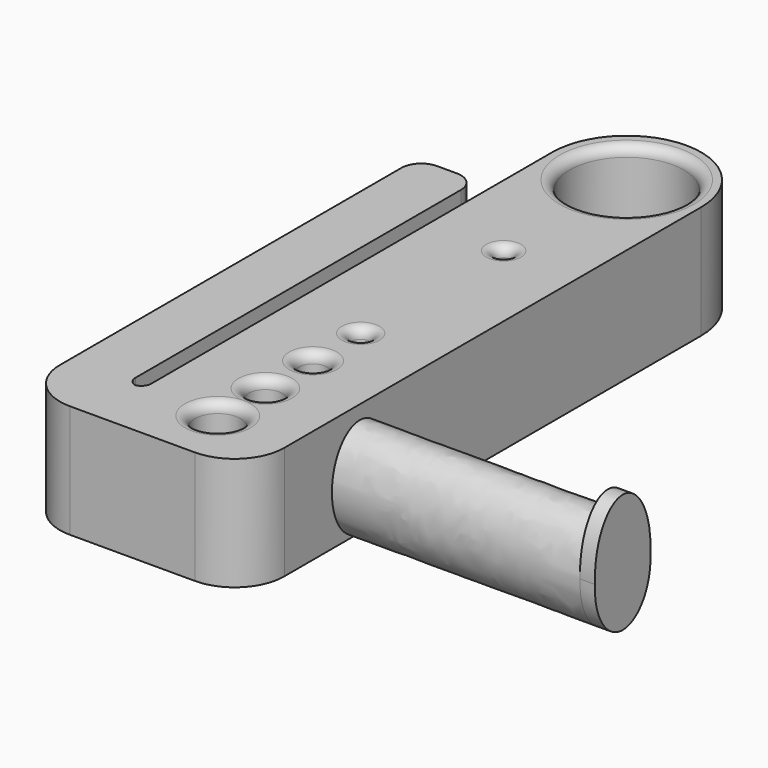
from build123d import *

# Parameters (mm, degrees)
F0_W        = 1.6
F0_H        = 6
F0_R        = 2.3
F0_R_2      = 1.7
F0_R_3      = 1.4
F0_R_4      = 0.9
F0_R_5      = 0.75
F0_R_6      = 5.75
F1_DEPTH    = 11.4
F2_R        = 5
F3_R        = 7.49999
F4_R        = 2
F5_T1_DEPTH = 11.4
F6_R        = 1
F8_DEPTH    = 25
F10_DEPTH   = 1.5


# Not quite as in the source:
# - a fillet or chamfer that OpenCascade refuses, or shapes differently, is made with other operations: its cross-section is extruded or revolved along the edge and cut away or added
# - a fillet or chamfer is up to 0.001 mm smaller than in the source, because OpenCascade refuses the exact size


with BuildPart() as f1:
    # F0 (on Top) → F1 (new body)
    with BuildSketch(Plane.XY):
        Polygon((6, 0), (0, 0), (0, -50), (6, -50), (6, -44), align=None)
        with Locations((6.8, -47)):
            Rectangle(F0_W, F0_H)
        Polygon((7.6, 15), (7.6, -44), (7.6, -50), (22.6, -50), (22.6, 15), align=None)
        with Locations((15.1, -44)):
            Circle(F0_R, mode=Mode.SUBTRACT)
        with Locations((15.1, -38)):
            Circle(F0_R_2, mode=Mode.SUBTRACT)
        with Locations((15.1, -32)):
            Circle(F0_R_3, mode=Mode.SUBTRACT)
        with Locations((15.1, -26)):
            Circle(F0_R_4, mode=Mode.SUBTRACT)
        with Locations((15.1, -8)):
            Circle(F0_R_5, mode=Mode.SUBTRACT)
        with Locations((15.1, 7.5)):
            Circle(F0_R_6, mode=Mode.SUBTRACT)
    extrude(amount=F1_DEPTH)

    # F2
    f2_edges = [f1.edges().sort_by_distance(p)[0] for p in [
        (0, -50, 5.7),
        (22.6, -50, 5.7),
    ]]
    fillet(f2_edges, radius=F2_R)

    # F3 (radius 7.5 in the source; OpenCascade refuses exactly that, so slightly less here)
    f3_edges = [f1.edges().sort_by_distance(p)[0] for p in [
        (22.6, 15, 5.7),
        (7.6, 15, 5.7),
    ]]
    fillet(f3_edges, radius=F3_R)

    # F4
    f4_edges = [f1.edges().sort_by_distance(p)[0] for p in [
        (0, 0, 5.7),
        (6, 0, 5.7),
    ]]
    fillet(f4_edges, radius=F4_R)

    # F5: fillet of radius 1 on 7 edges, made by hand

    # F5_s2 → F5_t1 (join)
    with BuildSketch(Plane.XY):
        with BuildLine():
            ThreePointArc((6, -43), (6.2928932188, -43.7071067812), (7, -44))
            Line((7, -44), (6, -44))
            Line((6, -44), (6, -43))
        make_face()
        with BuildLine():
            ThreePointArc((6.6, -44), (7.3071067812, -43.7071067812), (7.6, -43))
            Line((7.6, -43), (7.6, -44))
            Line((7.6, -44), (6.6, -44))
        make_face()
    extrude(amount=F5_T1_DEPTH)

    # F5_s3 → F5_t4 (revolve, cut)
    with BuildSketch(Plane.XZ.offset(44)):
        with BuildLine():
            ThreePointArc((17.4, 10.4), (17.6928932188, 11.1071067812), (18.4, 11.4))
            Line((18.4, 11.4), (17.4, 11.4))
            Line((17.4, 11.4), (17.4, 10.4))
        make_face()
    revolve(axis=Axis((15.1, -44, 11.4), (0, 0, 1)), mode=Mode.SUBTRACT)

    # F5_s5 → F5_t6 (revolve, cut)
    with BuildSketch(Plane.XZ.offset(38)):
        with BuildLine():
            ThreePointArc((16.8, 10.4), (17.0928932188, 11.1071067812), (17.8, 11.4))
            Line((17.8, 11.4), (16.8, 11.4))
            Line((16.8, 11.4), (16.8, 10.4))
        make_face()
    revolve(axis=Axis((15.1, -38, 11.4), (0, 0, 1)), mode=Mode.SUBTRACT)

    # F5_s7 → F5_t8 (revolve, cut)
    with BuildSketch(Plane.XZ.offset(32)):
        with BuildLine():
            ThreePointArc((16.5, 10.4), (16.7928932188, 11.1071067812), (17.5, 11.4))
            Line((17.5, 11.4), (16.5, 11.4))
            Line((16.5, 11.4), (16.5, 10.4))
        make_face()
    revolve(axis=Axis((15.1, -32, 11.4), (0, 0, 1)), mode=Mode.SUBTRACT)

    # F5_s9 → F5_t10 (revolve, cut)
    with BuildSketch(Plane.XZ.offset(26)):
        with BuildLine():
            ThreePointArc((16, 10.4), (16.2928932188, 11.1071067812), (17, 11.4))
            Line((17, 11.4), (16, 11.4))
            Line((16, 11.4), (16, 10.4))
        make_face()
    revolve(axis=Axis((15.1, -26, 11.4), (0, 0, 1)), mode=Mode.SUBTRACT)

    # F5_s11 → F5_t12 (revolve, cut)
    with BuildSketch(Plane.XZ.offset(8)):
        with BuildLine():
            ThreePointArc((15.85, 10.4), (16.1428932188, 11.1071067812), (16.85, 11.4))
            Line((16.85, 11.4), (15.85, 11.4))
            Line((15.85, 11.4), (15.85, 10.4))
        make_face()
    revolve(axis=Axis((15.1, -8, 11.4), (0, 0, 1)), mode=Mode.SUBTRACT)

    # F6
    f6_edges = [f1.edges().sort_by_distance(p)[0] for p in [
        (9.35, 7.5, 11.4),
    ]]
    fillet(f6_edges, radius=F6_R)

    # F7 (on face) → F8 (join)
    with BuildSketch(Plane.YZ.offset(22.6)):
        with BuildLine():
            add(Edge.make_bspline(
                [(-35.5, 0), (-29.4378221735, 0), (-32.4689110868, 7.5), (-35.5, 15), (-38.5310889132, 7.5), (-41.5621778265, 0), (-35.5, 0)],
                knots=[0, 0, 0, 2.0943951024, 2.0943951024, 4.1887902048, 4.1887902048, 6.2831853072, 6.2831853072, 6.2831853072], degree=2, weights=[1, 0.5, 1, 0.5, 1, 0.5, 1]))
        make_face()
    extrude(amount=F8_DEPTH)

    # F9 (on face) → F10 (join)
    with BuildSketch(Plane.YZ.offset(47.6)):
        with BuildLine():
            add(Edge.make_bspline(
                [(-38.9855071841, 5.4545454545), (-38.6950482521, 0), (-35.5, 0)],
                knots=[4.8034237584, 4.8034237584, 4.8034237584, 6.2831853072, 6.2831853072, 6.2831853072], degree=2, weights=[1, 0.7385489459, 1]))
            add(Edge.make_bspline(
                [(-35.5, 0), (-32.3049517479, 0), (-32.0144928159, 5.4545454545)],
                knots=[0, 0, 0, 1.4797615488, 1.4797615488, 1.4797615488], degree=2, weights=[1, 0.7385489459, 1]))
            add(Edge.make_bspline(
                [(-32.0144928159, 5.4545454545), (-32.0844033191, 6.548590015), (-32.4689110868, 7.5), (-35.5, 15), (-38.5310889132, 7.5), (-38.9155966809, 6.548590015), (-38.9855071841, 5.4545454545)],
                knots=[1.6228457594, 1.6228457594, 1.6228457594, 2.0943951024, 2.0943951024, 4.1887902048, 4.1887902048, 4.6603395478, 4.6603395478, 4.6603395478], degree=2, weights=[0.8255434974, 0.8874258867, 1, 0.5, 1, 0.8874258867, 0.8255434974]))
        make_face()
        with BuildLine():
            add(Edge.make_bspline(
                [(-38.9855071841, 5.4545454545), (-39.3340579025, 0), (-35.5, 0)],
                knots=[4.6603395478, 4.6603395478, 4.6603395478, 6.2831853072, 6.2831853072, 6.2831853072], degree=2, weights=[0.8255434974, 0.6125741133, 1]))
            add(Edge.make_bspline(
                [(-38.9855071841, 5.4545454545), (-38.6950482521, 0), (-35.5, 0)],
                knots=[4.8034237584, 4.8034237584, 4.8034237584, 6.2831853072, 6.2831853072, 6.2831853072], degree=2, weights=[1, 0.7385489459, 1]))
        make_face()
        with BuildLine():
            add(Edge.make_bspline(
                [(-35.5, 0), (-32.3049517479, 0), (-32.0144928159, 5.4545454545)],
                knots=[0, 0, 0, 1.4797615488, 1.4797615488, 1.4797615488], degree=2, weights=[1, 0.7385489459, 1]))
            add(Edge.make_bspline(
                [(-35.5, 0), (-31.6659420975, 0), (-32.0144928159, 5.4545454545)],
                knots=[0, 0, 0, 1.6228457594, 1.6228457594, 1.6228457594], degree=2, weights=[1, 0.6125741133, 0.8255434974]))
        make_face()
        with BuildLine():
            add(Edge.make_bspline(
                [(-32.0144928159, 5.4545454545), (-32.0844033191, 6.548590015), (-32.4689110868, 7.5), (-35.5, 15), (-38.5310889132, 7.5), (-38.9155966809, 6.548590015), (-38.9855071841, 5.4545454545)],
                knots=[1.6228457594, 1.6228457594, 1.6228457594, 2.0943951024, 2.0943951024, 4.1887902048, 4.1887902048, 4.6603395478, 4.6603395478, 4.6603395478], degree=2, weights=[0.8255434974, 0.8874258867, 1, 0.5, 1, 0.8874258867, 0.8255434974]))
            add(Edge.make_bspline(
                [(-32.0144928159, 5.4545454545), (-31.6659420975, 12), (-35.5, 12), (-39.3340579025, 12), (-38.9855071841, 5.4545454545)],
                knots=[1.4797615488, 1.4797615488, 1.4797615488, 3.1415926536, 3.1415926536, 4.8034237584, 4.8034237584, 4.8034237584], degree=2, weights=[1, 0.6741998625, 1, 0.6741998625, 1]))
        make_face()
    extrude(amount=F10_DEPTH)


solid = f1.part
